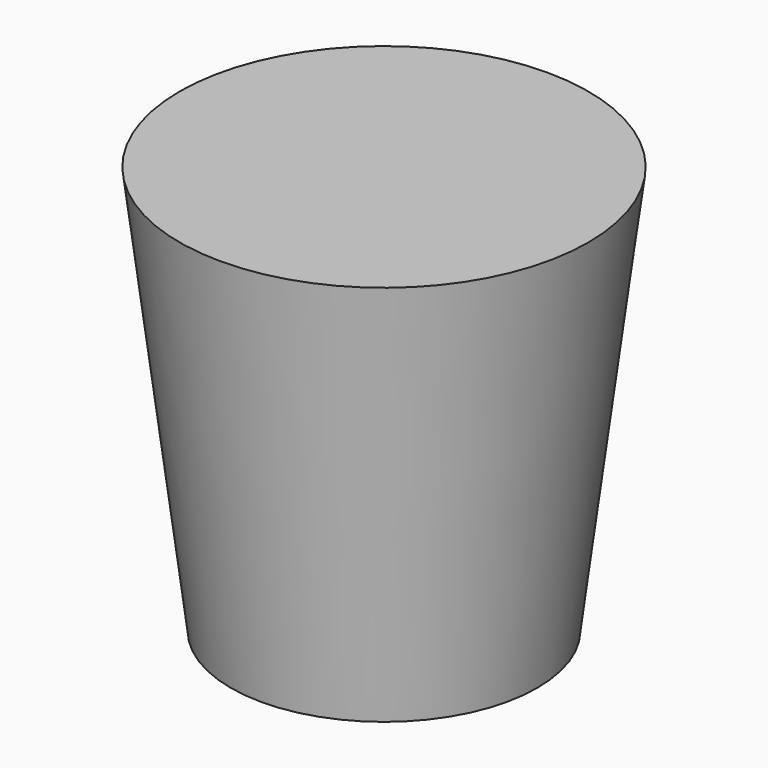
from build123d import *

# Parameters (mm, degrees)
F0_R     = 20
F1_DEPTH = 40
F2_SIZE2 = 4.99999
F2_SIZE  = 39.99999


# Not quite as in the source:
# - a fillet or chamfer is up to 0.001 mm smaller than in the source, because OpenCascade refuses the exact size


with BuildPart() as f1:
    # F0 (on Top) → F1 (new body)
    with BuildSketch(Plane.XY):
        Circle(F0_R)
    extrude(amount=F1_DEPTH)

    # F2 (size 40 and 5 in the source; OpenCascade refuses exactly that, so slightly less here)
    f2_edges = [f1.edges().sort_by_distance(p)[0] for p in [
        (-20, 0, 0),
    ]]
    f2_side = f1.faces().sort_by_distance((-20, 0, 20))[0]
    chamfer(f2_edges, length=F2_SIZE, length2=F2_SIZE2, reference=f2_side)


solid = f1.part
